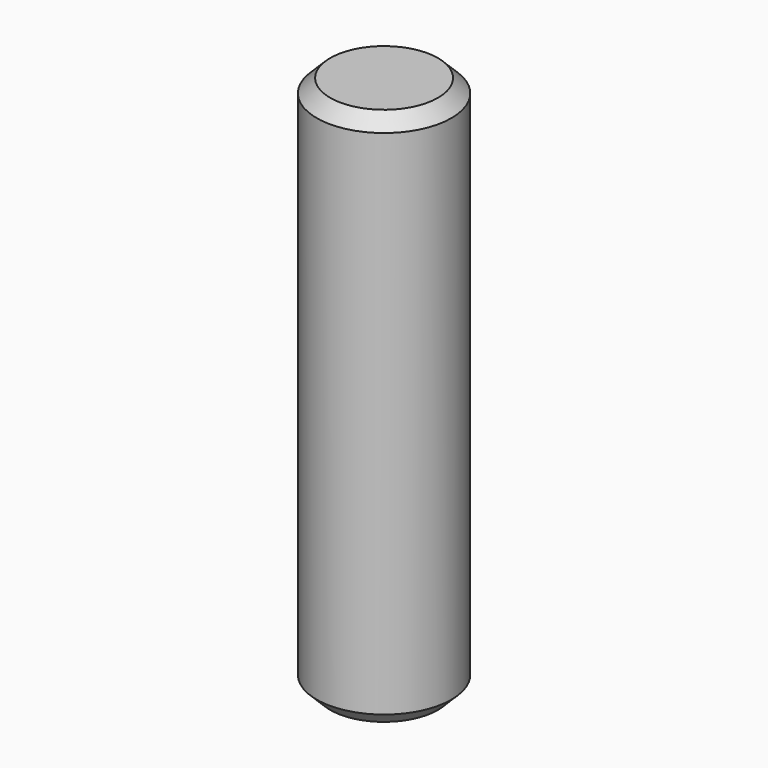
from build123d import *

# Parameters (mm, degrees)
F0_R     = 5
F1_DEPTH = 40
F2_SIZE  = 1


with BuildPart() as f1:
    # F0 (on Top) → F1 (new body)
    with BuildSketch(Plane.XY):
        with Locations((252.2108852863, -177.7984052896)):
            Circle(F0_R)
    extrude(amount=F1_DEPTH)

    # F2
    f2_edges = [f1.edges().sort_by_distance(p)[0] for p in [
        (247.210885, -177.798405, 40),
        (247.210885, -177.798405, 0),
    ]]
    chamfer(f2_edges, length=F2_SIZE)


solid = f1.part
